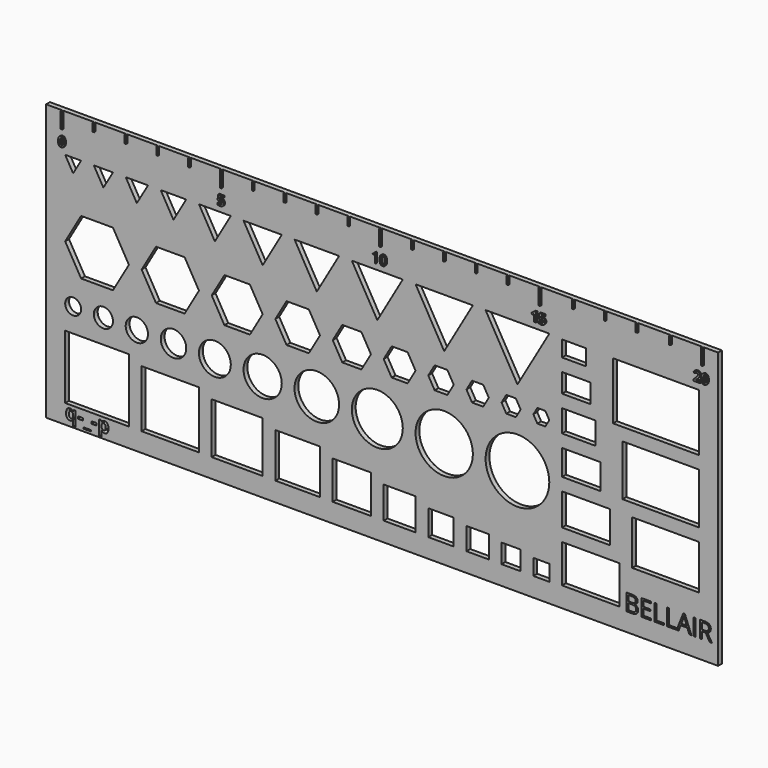
from build123d import *

# Parameters (mm, degrees)
F0_W         = 211
F0_H         = 86.6147367097
F0_W_2       = 20
F0_H_2       = 20
F0_W_3       = 18
F0_H_3       = 18
F0_W_4       = 16
F0_H_4       = 16
F0_W_5       = 14
F0_H_5       = 14
F0_W_6       = 12
F0_H_6       = 12
F0_R         = 2.5
F0_R_2       = 3
F0_R_3       = 3.5
F0_R_4       = 4
F0_R_5       = 5
F0_R_6       = 6
F0_R_7       = 7
F0_R_8       = 8
F0_W_7       = 8
F0_H_7       = 8
F0_W_8       = 7
F0_H_8       = 7
F0_W_9       = 6
F0_H_9       = 6
F0_W_10      = 5
F0_H_10      = 5
F0_W_11      = 10
F0_H_11      = 10
F0_R_9       = 9
F0_R_10      = 10
F0_W_12      = 15
F0_W_13      = 21
F0_W_14      = 10.5
F0_W_15      = 24
F0_W_16      = 9
F0_W_17      = 7.5
F0_W_18      = 27
F1_DEPTH     = 1.5
F2_TEXT_SIZE = 7.3304426082
F3_DEPTH     = 2
F4_TEXT_SIZE = 5.9722222222
F5_DEPTH     = 2
F6_W         = 0.5
F6_H         = 5
F6_H_2       = 2.5
F7_DEPTH     = 0.5


# Not quite as in the source:
# - Text() gives the source's letters only with a copy of the font that has no kerning and outlines rounded to 1/6400 em; it was checked with that copy


with BuildPart() as f1:
    # F0 (on Front) → F1 (new body)
    with BuildSketch(Plane.XZ):
        with Locations((99.5, 37.3073683549)):
            Rectangle(F0_W, F0_H)
        with Locations((10, 10)):
            Rectangle(F0_W_2, F0_H_2, mode=Mode.SUBTRACT)
        with Locations((33, 9)):
            Rectangle(F0_W_3, F0_H_3, mode=Mode.SUBTRACT)
        with Locations((54, 8)):
            Rectangle(F0_W_4, F0_H_4, mode=Mode.SUBTRACT)
        with Locations((73, 7)):
            Rectangle(F0_W_5, F0_H_5, mode=Mode.SUBTRACT)
        with Locations((90, 6)):
            Rectangle(F0_W_6, F0_H_6, mode=Mode.SUBTRACT)
        with Locations((2.5, 27.5)):
            Circle(F0_R, mode=Mode.SUBTRACT)
        with Locations((12, 27.5)):
            Circle(F0_R_2, mode=Mode.SUBTRACT)
        with Locations((22.5, 27.5)):
            Circle(F0_R_3, mode=Mode.SUBTRACT)
        with Locations((34, 27.5)):
            Circle(F0_R_4, mode=Mode.SUBTRACT)
        with Locations((47, 27.5)):
            Circle(F0_R_5, mode=Mode.SUBTRACT)
        with Locations((62, 27.5)):
            Circle(F0_R_6, mode=Mode.SUBTRACT)
        with Locations((79, 27.5)):
            Circle(F0_R_7, mode=Mode.SUBTRACT)
        with Locations((98, 27.5)):
            Circle(F0_R_8, mode=Mode.SUBTRACT)
        with Locations((118, 4)):
            Rectangle(F0_W_7, F0_H_7, mode=Mode.SUBTRACT)
        with Locations((129.5, 3.5)):
            Rectangle(F0_W_8, F0_H_8, mode=Mode.SUBTRACT)
        with Locations((140, 3)):
            Rectangle(F0_W_9, F0_H_9, mode=Mode.SUBTRACT)
        with Locations((149.5, 2.5)):
            Rectangle(F0_W_10, F0_H_10, mode=Mode.SUBTRACT)
        with Locations((105, 5)):
            Rectangle(F0_W_11, F0_H_11, mode=Mode.SUBTRACT)
        with Locations((165, 6.3147367097)):
            Rectangle(F0_W_3, F0_H_6, mode=Mode.SUBTRACT)
        with Locations((119, 27.5)):
            Circle(F0_R_9, mode=Mode.SUBTRACT)
        with Locations((142, 27.5)):
            Circle(F0_R_10, mode=Mode.SUBTRACT)
        with Locations((163.5, 21.3147367097)):
            Rectangle(F0_W_12, F0_H_11, mode=Mode.SUBTRACT)
        with Locations((188.5, 19.3147367097)):
            Rectangle(F0_W_13, F0_H_5, mode=Mode.SUBTRACT)
        with Locations((162, 34.3147367097)):
            Rectangle(F0_W_6, F0_H_7, mode=Mode.SUBTRACT)
        Polygon((0, 44.6961524227), (5, 53.3564064606), (15, 53.3564064606), (20, 44.6961524227), (15, 36.0358983849), (5, 36.0358983849), align=None, mode=Mode.SUBTRACT)
        Polygon((42, 44.6961524227), (37.5, 36.9019237886), (28.5, 36.9019237886), (24, 44.6961524227), (28.5, 52.4903810568), (37.5, 52.4903810568), align=None, mode=Mode.SUBTRACT)
        Polygon((46, 44.6961524227), (50, 51.624355653), (58, 51.624355653), (62, 44.6961524227), (58, 37.7679491924), (50, 37.7679491924), align=None, mode=Mode.SUBTRACT)
        Polygon((66, 44.6961524227), (69.5, 50.7583302492), (76.5, 50.7583302492), (80, 44.6961524227), (76.5, 38.6339745962), (69.5, 38.6339745962), align=None, mode=Mode.SUBTRACT)
        Polygon((84, 44.6961524227), (87, 49.8923048454), (93, 49.8923048454), (96, 44.6961524227), (93, 39.5), (87, 39.5), align=None, mode=Mode.SUBTRACT)
        Polygon((2.5, 64.2846096908), (0, 68.6147367097), (5, 68.6147367097), align=None, mode=Mode.SUBTRACT)
        Polygon((12, 63.418584287), (9, 68.6147367097), (15, 68.6147367097), align=None, mode=Mode.SUBTRACT)
        Polygon((22.5, 62.5525588833), (19, 68.6147367097), (26, 68.6147367097), align=None, mode=Mode.SUBTRACT)
        Polygon((34, 61.6865334795), (30, 68.6147367097), (38, 68.6147367097), align=None, mode=Mode.SUBTRACT)
        Polygon((47, 59.9544826719), (42, 68.6147367097), (52, 68.6147367097), align=None, mode=Mode.SUBTRACT)
        Polygon((62, 58.2224318643), (56, 68.6147367097), (68, 68.6147367097), align=None, mode=Mode.SUBTRACT)
        Polygon((79, 56.4903810568), (72, 68.6147367097), (86, 68.6147367097), align=None, mode=Mode.SUBTRACT)
        Polygon((98, 54.7583302492), (90, 68.6147367097), (106, 68.6147367097), align=None, mode=Mode.SUBTRACT)
        Polygon((100, 44.6961524227), (102.5, 49.0262794416), (107.5, 49.0262794416), (110, 44.6961524227), (107.5, 40.3660254038), (102.5, 40.3660254038), align=None, mode=Mode.SUBTRACT)
        Polygon((114, 44.6961524227), (116, 48.1602540378), (120, 48.1602540378), (122, 44.6961524227), (120, 41.2320508076), (116, 41.2320508076), align=None, mode=Mode.SUBTRACT)
        Polygon((126, 44.6961524227), (127.75, 47.727241336), (131.25, 47.727241336), (133, 44.6961524227), (131.25, 41.6650635095), (127.75, 41.6650635095), align=None, mode=Mode.SUBTRACT)
        Polygon((137, 44.6961524227), (138.5, 47.2942286341), (141.5, 47.2942286341), (143, 44.6961524227), (141.5, 42.0980762114), (138.5, 42.0980762114), align=None, mode=Mode.SUBTRACT)
        Polygon((147, 44.6961524227), (148.25, 46.8612159322), (150.75, 46.8612159322), (152, 44.6961524227), (150.75, 42.5310889132), (148.25, 42.5310889132), align=None, mode=Mode.SUBTRACT)
        with Locations((161.25, 45.8147367097)):
            Rectangle(F0_W_14, F0_H_8, mode=Mode.SUBTRACT)
        with Locations((187, 38.3147367097)):
            Rectangle(F0_W_15, F0_H_4, mode=Mode.SUBTRACT)
        with Locations((160.5, 56.3147367097)):
            Rectangle(F0_W_16, F0_H_9, mode=Mode.SUBTRACT)
        Polygon((119, 53.0262794416), (110, 68.6147367097), (128, 68.6147367097), align=None, mode=Mode.SUBTRACT)
        Polygon((142, 51.2942286341), (132, 68.6147367097), (152, 68.6147367097), align=None, mode=Mode.SUBTRACT)
        with Locations((159.75, 65.8147367097)):
            Rectangle(F0_W_17, F0_H_10, mode=Mode.SUBTRACT)
        with Locations((185.5, 59.3147367097)):
            Rectangle(F0_W_18, F0_H_3, mode=Mode.SUBTRACT)
    extrude(amount=F1_DEPTH)

    # F2 (on face) → F3 (cut)
    with BuildSketch(Plane.XZ.offset(1.5)):
        with Locations((175.5508746406, -0.2779186779)):
            Text('BELLAIR', F2_TEXT_SIZE, font='Open Sans', text_align=(TextAlign.LEFT, TextAlign.BOTTOM))
    extrude(amount=-F3_DEPTH, mode=Mode.SUBTRACT)

    # F4 (on face) → F5 (cut)
    with BuildSketch(Plane.XZ.offset(1.5)):
        with Locations((0, -4.3)):
            Text('q-_-p', F4_TEXT_SIZE, font='Open Sans', font_style=FontStyle.BOLD, text_align=(TextAlign.LEFT, TextAlign.BOTTOM))
    extrude(amount=-F5_DEPTH, mode=Mode.SUBTRACT)

    # F6 (on face) → F7 (join)
    with BuildSketch(Plane.XZ.offset(1.5)):
        with Locations((-0.75, 78.1147367097)):
            Rectangle(F6_W, F6_H)
        with Locations((9.25, 79.3647367097)):
            Rectangle(F6_W, F6_H_2)
        with Locations((19.25, 79.3647367097)):
            Rectangle(F6_W, F6_H_2)
        with Locations((29.25, 79.3647367097)):
            Rectangle(F6_W, F6_H_2)
        with Locations((39.25, 79.3647367097)):
            Rectangle(F6_W, F6_H_2)
        with Locations((49.25, 78.1147367097)):
            Rectangle(F6_W, F6_H)
        with Locations((59.25, 79.3647367097)):
            Rectangle(F6_W, F6_H_2)
        with Locations((69.25, 79.3647367097)):
            Rectangle(F6_W, F6_H_2)
        with Locations((79.25, 79.3647367097)):
            Rectangle(F6_W, F6_H_2)
        with Locations((89.25, 79.3647367097)):
            Rectangle(F6_W, F6_H_2)
        with Locations((99.25, 78.1147367097)):
            Rectangle(F6_W, F6_H)
        with Locations((109.25, 79.3647367097)):
            Rectangle(F6_W, F6_H_2)
        with Locations((119.25, 79.3647367097)):
            Rectangle(F6_W, F6_H_2)
        with Locations((129.25, 79.3647367097)):
            Rectangle(F6_W, F6_H_2)
        with Locations((139.25, 79.3647367097)):
            Rectangle(F6_W, F6_H_2)
        with Locations((149.25, 78.1147367097)):
            Rectangle(F6_W, F6_H)
        with Locations((159.75, 79.3647367097)):
            Rectangle(F6_W, F6_H_2)
        with Locations((169.75, 79.3647367097)):
            Rectangle(F6_W, F6_H_2)
        with Locations((179.75, 79.3647367097)):
            Rectangle(F6_W, F6_H_2)
        with Locations((190.25, 79.3647367097)):
            Rectangle(F6_W, F6_H_2)
        with Locations((200.25, 78.1147367097)):
            Rectangle(F6_W, F6_H)
        with BuildLine():
            Line((97.625, 72.7345283764), (97.625, 70.6147367097))
            Line((97.625, 70.6147367097), (97.9544270833, 70.6147367097))
            Line((97.9544270833, 70.6147367097), (97.9544270833, 73.5893460847))
            Line((97.9544270833, 73.5893460847), (97.669921875, 73.5893460847))
            Line((97.669921875, 73.5893460847), (96.8828125, 72.9806221264))
            Line((96.8828125, 72.9806221264), (97.0618489583, 72.7488512931))
            add(Edge.make_bspline(
                [(97.5458984375, 73.1456611889), (97.4928385417, 73.0991117097), (97.0618489583, 72.7488512931)],
                knots=[0, 0, 0, 1, 1, 1], degree=2))
            add(Edge.make_bspline(
                [(97.6412760417, 73.2351794181), (97.5989583333, 73.1922106681), (97.5458984375, 73.1456611889)],
                knots=[0, 0, 0, 1, 1, 1], degree=2))
            add(Edge.make_bspline(
                [(97.625, 72.7345283764), (97.625, 72.9995023347), (97.6412760417, 73.2351794181)],
                knots=[0, 0, 0, 1, 1, 1], degree=2))
        make_face()
        with BuildLine():
            add(Edge.make_bspline(
                [(-0.4905257889, 70.6147367097), (-0.6360782294, 70.5737210847), (-0.8118489583, 70.5737210847)],
                knots=[0.6691374514, 0.6691374514, 0.6691374514, 1, 1, 1], degree=2))
            Line((-0.4905257889, 70.6147367097), (-1.1203766284, 70.6147367097))
            add(Edge.make_bspline(
                [(-0.8118489583, 70.5737210847), (-0.9795602563, 70.5737210847), (-1.1203766284, 70.6147367097)],
                knots=[0, 0, 0, 0.3256694736, 0.3256694736, 0.3256694736], degree=2))
        make_face()
        with BuildLine():
            Line((-1.1203766284, 70.6147367097), (-0.4905257889, 70.6147367097))
            add(Edge.make_bspline(
                [(-0.025390625, 70.9483955639), (-0.1961600787, 70.6976868378), (-0.4905257889, 70.6147367097)],
                knots=[0, 0, 0, 0.6691374514, 0.6691374514, 0.6691374514], degree=2))
            add(Edge.make_bspline(
                [(0.2298177083, 72.1017158764), (0.2298177083, 71.3230700431), (-0.025390625, 70.9483955639)],
                knots=[0, 0, 0, 1, 1, 1], degree=2))
            add(Edge.make_bspline(
                [(-0.0335286458, 73.2455960847), (0.2298177083, 72.8549710847), (0.2298177083, 72.1017158764)],
                knots=[0, 0, 0, 1, 1, 1], degree=2))
            add(Edge.make_bspline(
                [(-0.8118489583, 73.6362210847), (-0.296875, 73.6362210847), (-0.0335286458, 73.2455960847)],
                knots=[0, 0, 0, 1, 1, 1], degree=2))
            add(Edge.make_bspline(
                [(-1.5950520833, 73.2628486889), (-1.3404947917, 73.6362210847), (-0.8118489583, 73.6362210847)],
                knots=[0, 0, 0, 1, 1, 1], degree=2))
            add(Edge.make_bspline(
                [(-1.849609375, 72.1017158764), (-1.849609375, 72.8894762931), (-1.5950520833, 73.2628486889)],
                knots=[0, 0, 0, 1, 1, 1], degree=2))
            add(Edge.make_bspline(
                [(-1.5882161458, 70.9604398347), (-1.849609375, 71.3471585847), (-1.849609375, 72.1017158764)],
                knots=[0, 0, 0, 1, 1, 1], degree=2))
            add(Edge.make_bspline(
                [(-1.1203766284, 70.6147367097), (-1.411950712, 70.6996635765), (-1.5882161458, 70.9604398347)],
                knots=[0.3256694736, 0.3256694736, 0.3256694736, 1, 1, 1], degree=2))
        make_face()
        with BuildLine():
            add(Edge.make_bspline(
                [(-1.224609375, 72.1017158764), (-1.224609375, 71.5548408764), (-1.1302083333, 71.3178617097)],
                knots=[0, 0, 0, 1, 1, 1], degree=2))
            add(Edge.make_bspline(
                [(-1.1292317708, 72.8881742097), (-1.224609375, 72.6492419181), (-1.224609375, 72.1017158764)],
                knots=[0, 0, 0, 1, 1, 1], degree=2))
            add(Edge.make_bspline(
                [(-0.8118489583, 73.1271065014), (-1.0338541667, 73.1271065014), (-1.1292317708, 72.8881742097)],
                knots=[0, 0, 0, 1, 1, 1], degree=2))
            add(Edge.make_bspline(
                [(-0.4954427083, 72.8881742097), (-0.5944010417, 73.1271065014), (-0.8118489583, 73.1271065014)],
                knots=[0, 0, 0, 1, 1, 1], degree=2))
            add(Edge.make_bspline(
                [(-0.396484375, 72.1017158764), (-0.396484375, 72.6492419181), (-0.4954427083, 72.8881742097)],
                knots=[0, 0, 0, 1, 1, 1], degree=2))
            add(Edge.make_bspline(
                [(-0.494140625, 71.3207913972), (-0.396484375, 71.5607002514), (-0.396484375, 72.1017158764)],
                knots=[0, 0, 0, 1, 1, 1], degree=2))
            add(Edge.make_bspline(
                [(-0.8118489583, 71.0808825431), (-0.591796875, 71.0808825431), (-0.494140625, 71.3207913972)],
                knots=[0, 0, 0, 1, 1, 1], degree=2))
            add(Edge.make_bspline(
                [(-1.1302083333, 71.3178617097), (-1.0358072917, 71.0808825431), (-0.8118489583, 71.0808825431)],
                knots=[0, 0, 0, 1, 1, 1], degree=2))
        make_face(mode=Mode.SUBTRACT)
        with BuildLine():
            add(Edge.make_bspline(
                [(49.411395169, 70.6147367097), (49.2284619736, 70.5737210847), (49.0052083333, 70.5737210847)],
                knots=[0.6094332671, 0.6094332671, 0.6094332671, 1, 1, 1], degree=2))
            Line((49.411395169, 70.6147367097), (48.5524472231, 70.6147367097))
            add(Edge.make_bspline(
                [(49.0052083333, 70.5737210847), (48.7543346418, 70.5737210847), (48.5524472231, 70.6147367097)],
                knots=[0, 0, 0, 0.5050353738, 0.5050353738, 0.5050353738], degree=2))
        make_face()
        with BuildLine():
            Line((48.5524472231, 70.6147367097), (49.411395169, 70.6147367097))
            add(Edge.make_bspline(
                [(49.8841145833, 70.8426012931), (49.696840819, 70.6787367493), (49.411395169, 70.6147367097)],
                knots=[0, 0, 0, 0.6094332671, 0.6094332671, 0.6094332671], degree=2))
            add(Edge.make_bspline(
                [(50.19140625, 71.6095283764), (50.19140625, 71.1114815014), (49.8841145833, 70.8426012931)],
                knots=[0, 0, 0, 1, 1, 1], degree=2))
            add(Edge.make_bspline(
                [(49.9358723958, 72.2729398347), (50.19140625, 72.0307523347), (50.19140625, 71.6095283764)],
                knots=[0, 0, 0, 1, 1, 1], degree=2))
            add(Edge.make_bspline(
                [(49.2493489583, 72.5151273347), (49.6803385417, 72.5151273347), (49.9358723958, 72.2729398347)],
                knots=[0, 0, 0, 1, 1, 1], degree=2))
            add(Edge.make_bspline(
                [(48.9420572917, 72.4864815014), (49.06640625, 72.5151273347), (49.2493489583, 72.5151273347)],
                knots=[0, 0, 0, 1, 1, 1], degree=2))
            Line((48.9420572917, 72.4864815014), (48.87109375, 72.4721585847))
            Line((48.87109375, 72.4721585847), (48.92578125, 73.0561429597))
            Line((48.92578125, 73.0561429597), (49.9876302083, 73.0561429597))
            Line((49.9876302083, 73.0561429597), (49.9876302083, 73.5893460847))
            Line((49.9876302083, 73.5893460847), (48.3743489583, 73.5893460847))
            Line((48.3743489583, 73.5893460847), (48.2623697917, 72.0737210847))
            Line((48.2623697917, 72.0737210847), (48.5130208333, 71.9389554597))
            add(Edge.make_bspline(
                [(48.724609375, 71.9851794181), (48.5944010417, 71.9636950431), (48.5130208333, 71.9389554597)],
                knots=[0, 0, 0, 1, 1, 1], degree=2))
            add(Edge.make_bspline(
                [(48.9622395833, 72.0066637931), (48.8548177083, 72.0066637931), (48.724609375, 71.9851794181)],
                knots=[0, 0, 0, 1, 1, 1], degree=2))
            add(Edge.make_bspline(
                [(49.55859375, 71.5567940014), (49.55859375, 72.0066637931), (48.9622395833, 72.0066637931)],
                knots=[0, 0, 0, 1, 1, 1], degree=2))
            add(Edge.make_bspline(
                [(48.982421875, 71.0847887931), (49.55859375, 71.0847887931), (49.55859375, 71.5567940014)],
                knots=[0, 0, 0, 1, 1, 1], degree=2))
            add(Edge.make_bspline(
                [(48.5777994792, 71.1388252514), (48.7916666667, 71.0847887931), (48.982421875, 71.0847887931)],
                knots=[0, 0, 0, 1, 1, 1], degree=2))
            add(Edge.make_bspline(
                [(48.2037760417, 71.2781481681), (48.3639322917, 71.1928617097), (48.5777994792, 71.1388252514)],
                knots=[0, 0, 0, 1, 1, 1], degree=2))
            Line((48.2037760417, 71.2781481681), (48.2037760417, 70.7345283764))
            add(Edge.make_bspline(
                [(48.5524472231, 70.6147367097), (48.3545855762, 70.6549344554), (48.2037760417, 70.7345283764)],
                knots=[0.5050353738, 0.5050353738, 0.5050353738, 1, 1, 1], degree=2))
        make_face()
        with BuildLine():
            add(Edge.make_bspline(
                [(200.7578785799, 70.6147367097), (200.4663044963, 70.6996635765), (200.2900390625, 70.9604398347)],
                knots=[0.3256694736, 0.3256694736, 0.3256694736, 1, 1, 1], degree=2))
            Line((200.7578785799, 70.6147367097), (201.3877294194, 70.6147367097))
            add(Edge.make_bspline(
                [(201.8528645833, 70.9483955639), (201.6820951296, 70.6976868378), (201.3877294194, 70.6147367097)],
                knots=[0, 0, 0, 0.6691374514, 0.6691374514, 0.6691374514], degree=2))
            add(Edge.make_bspline(
                [(202.1080729167, 72.1017158764), (202.1080729167, 71.3230700431), (201.8528645833, 70.9483955639)],
                knots=[0, 0, 0, 1, 1, 1], degree=2))
            add(Edge.make_bspline(
                [(201.8447265625, 73.2455960847), (202.1080729167, 72.8549710847), (202.1080729167, 72.1017158764)],
                knots=[0, 0, 0, 1, 1, 1], degree=2))
            add(Edge.make_bspline(
                [(201.06640625, 73.6362210847), (201.5813802083, 73.6362210847), (201.8447265625, 73.2455960847)],
                knots=[0, 0, 0, 1, 1, 1], degree=2))
            add(Edge.make_bspline(
                [(200.283203125, 73.2628486889), (200.5377604167, 73.6362210847), (201.06640625, 73.6362210847)],
                knots=[0, 0, 0, 1, 1, 1], degree=2))
            add(Edge.make_bspline(
                [(200.0286458333, 72.1017158764), (200.0286458333, 72.8894762931), (200.283203125, 73.2628486889)],
                knots=[0, 0, 0, 1, 1, 1], degree=2))
            add(Edge.make_bspline(
                [(200.2900390625, 70.9604398347), (200.0286458333, 71.3471585847), (200.0286458333, 72.1017158764)],
                knots=[0, 0, 0, 1, 1, 1], degree=2))
        make_face()
        with BuildLine():
            add(Edge.make_bspline(
                [(200.6536458333, 72.1017158764), (200.6536458333, 71.5548408764), (200.748046875, 71.3178617097)],
                knots=[0, 0, 0, 1, 1, 1], degree=2))
            add(Edge.make_bspline(
                [(200.7490234375, 72.8881742097), (200.6536458333, 72.6492419181), (200.6536458333, 72.1017158764)],
                knots=[0, 0, 0, 1, 1, 1], degree=2))
            add(Edge.make_bspline(
                [(201.06640625, 73.1271065014), (200.8444010417, 73.1271065014), (200.7490234375, 72.8881742097)],
                knots=[0, 0, 0, 1, 1, 1], degree=2))
            add(Edge.make_bspline(
                [(201.3828125, 72.8881742097), (201.2838541667, 73.1271065014), (201.06640625, 73.1271065014)],
                knots=[0, 0, 0, 1, 1, 1], degree=2))
            add(Edge.make_bspline(
                [(201.4817708333, 72.1017158764), (201.4817708333, 72.6492419181), (201.3828125, 72.8881742097)],
                knots=[0, 0, 0, 1, 1, 1], degree=2))
            add(Edge.make_bspline(
                [(201.3841145833, 71.3207913972), (201.4817708333, 71.5607002514), (201.4817708333, 72.1017158764)],
                knots=[0, 0, 0, 1, 1, 1], degree=2))
            add(Edge.make_bspline(
                [(201.06640625, 71.0808825431), (201.2864583333, 71.0808825431), (201.3841145833, 71.3207913972)],
                knots=[0, 0, 0, 1, 1, 1], degree=2))
            add(Edge.make_bspline(
                [(200.748046875, 71.3178617097), (200.8424479167, 71.0808825431), (201.06640625, 71.0808825431)],
                knots=[0, 0, 0, 1, 1, 1], degree=2))
        make_face(mode=Mode.SUBTRACT)
        with BuildLine():
            Line((201.3877294194, 70.6147367097), (200.7578785799, 70.6147367097))
            add(Edge.make_bspline(
                [(201.06640625, 70.5737210847), (200.8986949521, 70.5737210847), (200.7578785799, 70.6147367097)],
                knots=[0, 0, 0, 0.3256694736, 0.3256694736, 0.3256694736], degree=2))
            add(Edge.make_bspline(
                [(201.3877294194, 70.6147367097), (201.2421769789, 70.5737210847), (201.06640625, 70.5737210847)],
                knots=[0.6691374514, 0.6691374514, 0.6691374514, 1, 1, 1], degree=2))
        make_face()
        with BuildLine():
            Line((197.6666666667, 71.0522367097), (197.6666666667, 70.6147367097))
            Line((197.6666666667, 70.6147367097), (199.74609375, 70.6147367097))
            Line((199.74609375, 70.6147367097), (199.74609375, 71.1440335847))
            Line((199.74609375, 71.1440335847), (198.4498697917, 71.1440335847))
            Line((198.4498697917, 71.1440335847), (198.4498697917, 71.1720283764))
            Line((198.4498697917, 71.1720283764), (198.8326822917, 71.5320544181))
            add(Edge.make_bspline(
                [(199.3665364583, 72.0714424389), (199.21484375, 71.8823148347), (198.8326822917, 71.5320544181)],
                knots=[0, 0, 0, 1, 1, 1], degree=2))
            add(Edge.make_bspline(
                [(199.5904947917, 72.4405830639), (199.5182291667, 72.2605700431), (199.3665364583, 72.0714424389)],
                knots=[0, 0, 0, 1, 1, 1], degree=2))
            add(Edge.make_bspline(
                [(199.6627604167, 72.8263252514), (199.6627604167, 72.6205960847), (199.5904947917, 72.4405830639)],
                knots=[0, 0, 0, 1, 1, 1], degree=2))
            add(Edge.make_bspline(
                [(199.5445963542, 73.2452705639), (199.6627604167, 73.0620023347), (199.6627604167, 72.8263252514)],
                knots=[0, 0, 0, 1, 1, 1], degree=2))
            add(Edge.make_bspline(
                [(199.212890625, 73.5301012931), (199.4264322917, 73.4285387931), (199.5445963542, 73.2452705639)],
                knots=[0, 0, 0, 1, 1, 1], degree=2))
            add(Edge.make_bspline(
                [(198.720703125, 73.6316637931), (198.9993489583, 73.6316637931), (199.212890625, 73.5301012931)],
                knots=[0, 0, 0, 1, 1, 1], degree=2))
            add(Edge.make_bspline(
                [(198.3382161458, 73.5899971264), (198.5091145833, 73.6316637931), (198.720703125, 73.6316637931)],
                knots=[0, 0, 0, 1, 1, 1], degree=2))
            add(Edge.make_bspline(
                [(198.0227864583, 73.4711820222), (198.1673177083, 73.5483304597), (198.3382161458, 73.5899971264)],
                knots=[0, 0, 0, 1, 1, 1], degree=2))
            add(Edge.make_bspline(
                [(197.6588541667, 73.2065335847), (197.8782552083, 73.3940335847), (198.0227864583, 73.4711820222)],
                knots=[0, 0, 0, 1, 1, 1], degree=2))
            Line((197.6588541667, 73.2065335847), (198.0006510417, 72.8015856681))
            add(Edge.make_bspline(
                [(198.3404947917, 73.0274971264), (198.177734375, 72.9480700431), (198.0006510417, 72.8015856681)],
                knots=[0, 0, 0, 1, 1, 1], degree=2))
            add(Edge.make_bspline(
                [(198.67578125, 73.1069242097), (198.5032552083, 73.1069242097), (198.3404947917, 73.0274971264)],
                knots=[0, 0, 0, 1, 1, 1], degree=2))
            add(Edge.make_bspline(
                [(198.939453125, 73.0193591056), (198.8404947917, 73.1069242097), (198.67578125, 73.1069242097)],
                knots=[0, 0, 0, 1, 1, 1], degree=2))
            add(Edge.make_bspline(
                [(199.0384114583, 72.7527575431), (199.0384114583, 72.9317940014), (198.939453125, 73.0193591056)],
                knots=[0, 0, 0, 1, 1, 1], degree=2))
            add(Edge.make_bspline(
                [(198.9934895833, 72.5209867097), (199.0384114583, 72.6329658764), (199.0384114583, 72.7527575431)],
                knots=[0, 0, 0, 1, 1, 1], degree=2))
            add(Edge.make_bspline(
                [(198.8470052083, 72.2778226472), (198.9485677083, 72.4090075431), (198.9934895833, 72.5209867097)],
                knots=[0, 0, 0, 1, 1, 1], degree=2))
            add(Edge.make_bspline(
                [(198.4134114583, 71.8067940014), (198.7454427083, 72.1466377514), (198.8470052083, 72.2778226472)],
                knots=[0, 0, 0, 1, 1, 1], degree=2))
            Line((198.4134114583, 71.8067940014), (197.6666666667, 71.0522367097))
        make_face()
        with BuildLine():
            add(Edge.make_bspline(
                [(149.4307024314, 70.6147367097), (149.2328407846, 70.6549344554), (149.08203125, 70.7345283764)],
                knots=[0.5050353738, 0.5050353738, 0.5050353738, 1, 1, 1], degree=2))
            Line((149.4307024314, 70.6147367097), (150.2896503774, 70.6147367097))
            add(Edge.make_bspline(
                [(150.7623697917, 70.8426012931), (150.5750960273, 70.6787367493), (150.2896503774, 70.6147367097)],
                knots=[0, 0, 0, 0.6094332671, 0.6094332671, 0.6094332671], degree=2))
            add(Edge.make_bspline(
                [(151.0696614583, 71.6095283764), (151.0696614583, 71.1114815014), (150.7623697917, 70.8426012931)],
                knots=[0, 0, 0, 1, 1, 1], degree=2))
            add(Edge.make_bspline(
                [(150.8141276042, 72.2729398347), (151.0696614583, 72.0307523347), (151.0696614583, 71.6095283764)],
                knots=[0, 0, 0, 1, 1, 1], degree=2))
            add(Edge.make_bspline(
                [(150.1276041667, 72.5151273347), (150.55859375, 72.5151273347), (150.8141276042, 72.2729398347)],
                knots=[0, 0, 0, 1, 1, 1], degree=2))
            add(Edge.make_bspline(
                [(149.8203125, 72.4864815014), (149.9446614583, 72.5151273347), (150.1276041667, 72.5151273347)],
                knots=[0, 0, 0, 1, 1, 1], degree=2))
            Line((149.8203125, 72.4864815014), (149.7493489583, 72.4721585847))
            Line((149.7493489583, 72.4721585847), (149.8040364583, 73.0561429597))
            Line((149.8040364583, 73.0561429597), (150.8658854167, 73.0561429597))
            Line((150.8658854167, 73.0561429597), (150.8658854167, 73.5893460847))
            Line((150.8658854167, 73.5893460847), (149.2526041667, 73.5893460847))
            Line((149.2526041667, 73.5893460847), (149.140625, 72.0737210847))
            Line((149.140625, 72.0737210847), (149.3912760417, 71.9389554597))
            add(Edge.make_bspline(
                [(149.6028645833, 71.9851794181), (149.47265625, 71.9636950431), (149.3912760417, 71.9389554597)],
                knots=[0, 0, 0, 1, 1, 1], degree=2))
            add(Edge.make_bspline(
                [(149.8404947917, 72.0066637931), (149.7330729167, 72.0066637931), (149.6028645833, 71.9851794181)],
                knots=[0, 0, 0, 1, 1, 1], degree=2))
            add(Edge.make_bspline(
                [(150.4368489583, 71.5567940014), (150.4368489583, 72.0066637931), (149.8404947917, 72.0066637931)],
                knots=[0, 0, 0, 1, 1, 1], degree=2))
            add(Edge.make_bspline(
                [(149.8606770833, 71.0847887931), (150.4368489583, 71.0847887931), (150.4368489583, 71.5567940014)],
                knots=[0, 0, 0, 1, 1, 1], degree=2))
            add(Edge.make_bspline(
                [(149.4560546875, 71.1388252514), (149.669921875, 71.0847887931), (149.8606770833, 71.0847887931)],
                knots=[0, 0, 0, 1, 1, 1], degree=2))
            add(Edge.make_bspline(
                [(149.08203125, 71.2781481681), (149.2421875, 71.1928617097), (149.4560546875, 71.1388252514)],
                knots=[0, 0, 0, 1, 1, 1], degree=2))
            Line((149.08203125, 71.2781481681), (149.08203125, 70.7345283764))
        make_face()
        with BuildLine():
            Line((150.2896503774, 70.6147367097), (149.4307024314, 70.6147367097))
            add(Edge.make_bspline(
                [(149.8834635417, 70.5737210847), (149.6325898501, 70.5737210847), (149.4307024314, 70.6147367097)],
                knots=[0, 0, 0, 0.5050353738, 0.5050353738, 0.5050353738], degree=2))
            add(Edge.make_bspline(
                [(150.2896503774, 70.6147367097), (150.106717182, 70.5737210847), (149.8834635417, 70.5737210847)],
                knots=[0.6094332671, 0.6094332671, 0.6094332671, 1, 1, 1], degree=2))
        make_face()
        with BuildLine():
            Line((147.5924479167, 72.3360908764), (147.5924479167, 70.6147367097))
            Line((147.5924479167, 70.6147367097), (148.2213541667, 70.6147367097))
            Line((148.2213541667, 70.6147367097), (148.2213541667, 73.5893460847))
            Line((148.2213541667, 73.5893460847), (147.7044270833, 73.5893460847))
            Line((147.7044270833, 73.5893460847), (146.74609375, 72.8263252514))
            Line((146.74609375, 72.8263252514), (147.0494791667, 72.4480700431))
            Line((147.0494791667, 72.4480700431), (147.3912760417, 72.7228096264))
            add(Edge.make_bspline(
                [(147.6087239583, 72.9278877514), (147.4524739583, 72.7716377514), (147.3912760417, 72.7228096264)],
                knots=[0, 0, 0, 1, 1, 1], degree=2))
            Line((147.6087239583, 72.9278877514), (147.5989583333, 72.6186429597))
            Line((147.5989583333, 72.6186429597), (147.5924479167, 72.3360908764))
        make_face()
        with BuildLine():
            add(Edge.make_bspline(
                [(99.7831227303, 70.6147367097), (99.5092784682, 70.7001397313), (99.3401692708, 70.9633695222)],
                knots=[0.3244428423, 0.3244428423, 0.3244428423, 1, 1, 1], degree=2))
            Line((99.7831227303, 70.6147367097), (100.3712922865, 70.6147367097))
            add(Edge.make_bspline(
                [(100.8141276042, 70.9542549389), (100.6507956148, 70.6986524013), (100.3712922865, 70.6147367097)],
                knots=[0, 0, 0, 0.6716946069, 0.6716946069, 0.6716946069], degree=2))
            add(Edge.make_bspline(
                [(101.0572916667, 72.1062731681), (101.0572916667, 71.3347887931), (100.8141276042, 70.9542549389)],
                knots=[0, 0, 0, 1, 1, 1], degree=2))
            add(Edge.make_bspline(
                [(100.8059895833, 73.2433174389), (101.0572916667, 72.8504137931), (101.0572916667, 72.1062731681)],
                knots=[0, 0, 0, 1, 1, 1], degree=2))
            add(Edge.make_bspline(
                [(100.0703125, 73.6362210847), (100.5546875, 73.6362210847), (100.8059895833, 73.2433174389)],
                knots=[0, 0, 0, 1, 1, 1], degree=2))
            add(Edge.make_bspline(
                [(99.33203125, 73.2595934806), (99.57421875, 73.6362210847), (100.0703125, 73.6362210847)],
                knots=[0, 0, 0, 1, 1, 1], degree=2))
            add(Edge.make_bspline(
                [(99.08984375, 72.1062731681), (99.08984375, 72.8829658764), (99.33203125, 73.2595934806)],
                knots=[0, 0, 0, 1, 1, 1], degree=2))
            add(Edge.make_bspline(
                [(99.3401692708, 70.9633695222), (99.08984375, 71.3530179597), (99.08984375, 72.1062731681)],
                knots=[0, 0, 0, 1, 1, 1], degree=2))
        make_face()
        with BuildLine():
            add(Edge.make_bspline(
                [(99.431640625, 72.1062731681), (99.431640625, 71.4571846264), (99.5843098958, 71.1609606681)],
                knots=[0, 0, 0, 1, 1, 1], degree=2))
            add(Edge.make_bspline(
                [(99.5843098958, 73.0493070222), (99.431640625, 72.7553617097), (99.431640625, 72.1062731681)],
                knots=[0, 0, 0, 1, 1, 1], degree=2))
            add(Edge.make_bspline(
                [(100.0703125, 73.3432523347), (99.7369791667, 73.3432523347), (99.5843098958, 73.0493070222)],
                knots=[0, 0, 0, 1, 1, 1], degree=2))
            add(Edge.make_bspline(
                [(100.5595703125, 73.0450752514), (100.408203125, 73.3432523347), (100.0703125, 73.3432523347)],
                knots=[0, 0, 0, 1, 1, 1], degree=2))
            add(Edge.make_bspline(
                [(100.7109375, 72.1062731681), (100.7109375, 72.7468981681), (100.5595703125, 73.0450752514)],
                knots=[0, 0, 0, 1, 1, 1], degree=2))
            add(Edge.make_bspline(
                [(100.5595703125, 71.1648669181), (100.7109375, 71.4649971264), (100.7109375, 72.1062731681)],
                knots=[0, 0, 0, 1, 1, 1], degree=2))
            add(Edge.make_bspline(
                [(100.0703125, 70.8647367097), (100.408203125, 70.8647367097), (100.5595703125, 71.1648669181)],
                knots=[0, 0, 0, 1, 1, 1], degree=2))
            add(Edge.make_bspline(
                [(99.5843098958, 71.1609606681), (99.7369791667, 70.8647367097), (100.0703125, 70.8647367097)],
                knots=[0, 0, 0, 1, 1, 1], degree=2))
        make_face(mode=Mode.SUBTRACT)
        with BuildLine():
            Line((100.3712922865, 70.6147367097), (99.7831227303, 70.6147367097))
            add(Edge.make_bspline(
                [(100.0703125, 70.5737210847), (99.9146390789, 70.5737210847), (99.7831227303, 70.6147367097)],
                knots=[0, 0, 0, 0.3244428423, 0.3244428423, 0.3244428423], degree=2))
            add(Edge.make_bspline(
                [(100.3712922865, 70.6147367097), (100.234678937, 70.5737210847), (100.0703125, 70.5737210847)],
                knots=[0.6716946069, 0.6716946069, 0.6716946069, 1, 1, 1], degree=2))
        make_face()
    extrude(amount=F7_DEPTH)


solid = f1.part
